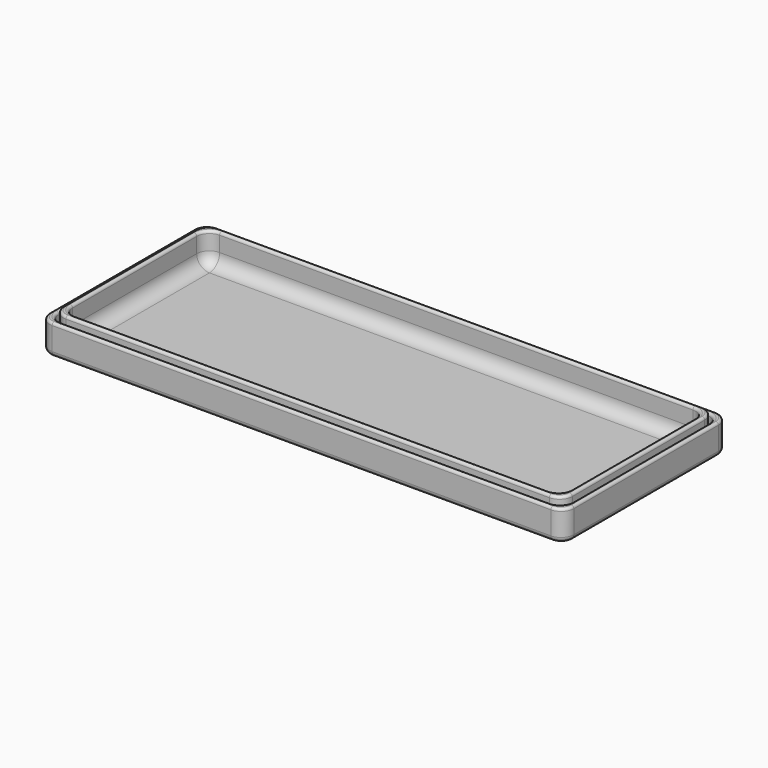
from build123d import *

# Parameters (mm, degrees)
F0_W     = 206
F0_H     = 81
F1_DEPTH = 2
F2_W     = 200
F2_H     = 75
F2_W_2   = 196
F2_H_2   = 71
F3_DEPTH = 12
F2_W_3   = 206
F2_H_3   = 81
F2_W_4   = 202
F2_H_4   = 77
F4_DEPTH = 10
F5_R     = 5
F6_R     = 5
F7_R     = 0.99999
F8_R     = 5
F9_R     = 5
F10_R    = 2
F11_R    = 0.99999
F12_R    = 5


# Not quite as in the source:
# - a fillet or chamfer is up to 0.001 mm smaller than in the source, because OpenCascade refuses the exact size


with BuildPart() as f1:
    # F0 (on Top) → F1 (new body)
    with BuildSketch(Plane.XY):
        Rectangle(F0_W, F0_H)
    extrude(amount=F1_DEPTH)

    # F2 (on face) → F3 (join)
    with BuildSketch(Plane.XY.offset(2)):
        Rectangle(F2_W, F2_H)
        Rectangle(F2_W_2, F2_H_2, mode=Mode.SUBTRACT)
    extrude(amount=F3_DEPTH)

    # F2 (on face) → F4 (join)
    with BuildSketch(Plane.XY.offset(2)):
        Rectangle(F2_W_3, F2_H_3)
        Rectangle(F2_W_4, F2_H_4, mode=Mode.SUBTRACT)
    extrude(amount=F4_DEPTH)

    # F5
    f5_edges = [f1.edges().sort_by_distance(p)[0] for p in [
        (-100, -37.5, 8),
        (-100, 37.5, 8),
        (100, 37.5, 8),
        (100, -37.5, 8),
    ]]
    fillet(f5_edges, radius=F5_R)

    # F6
    f6_edges = [f1.edges().sort_by_distance(p)[0] for p in [
        (-98, -35.5, 8),
        (-98, 35.5, 8),
        (98, 35.5, 8),
        (98, -35.5, 8),
    ]]
    fillet(f6_edges, radius=F6_R)

    # F7 (radius 1 in the source; OpenCascade refuses exactly that, so slightly less here)
    f7_edges = [f1.edges().sort_by_distance(p)[0] for p in [
        (-98, 0, 14),
        (-96.535534, -34.035534, 14),
        (-96.535534, 34.035534, 14),
        (0, -35.5, 14),
        (0, 35.5, 14),
        (96.535534, -34.035534, 14),
        (96.535534, 34.035534, 14),
        (98, 0, 14),
        (0, 37.5, 14),
        (98.535534, 36.035534, 14),
        (-98.535534, 36.035534, 14),
        (100, 0, 14),
        (-100, 0, 14),
        (98.535534, -36.035534, 14),
        (-98.535534, -36.035534, 14),
        (0, -37.5, 14),
    ]]
    fillet(f7_edges, radius=F7_R)

    # F8
    f8_edges = [f1.edges().sort_by_distance(p)[0] for p in [
        (-101, 38.5, 7),
        (-101, -38.5, 7),
        (101, -38.5, 7),
        (101, 38.5, 7),
    ]]
    fillet(f8_edges, radius=F8_R)

    # F9
    f9_edges = [f1.edges().sort_by_distance(p)[0] for p in [
        (-103, -40.5, 6),
        (103, -40.5, 6),
        (103, 40.5, 6),
        (-103, 40.5, 6),
    ]]
    fillet(f9_edges, radius=F9_R)

    # F10
    f10_edges = [f1.edges().sort_by_distance(p)[0] for p in [
        (0, -40.5, 0),
        (-101.535534, -39.035534, 0),
        (101.535534, -39.035534, 0),
        (-103, 0, 0),
        (103, 0, 0),
        (-101.535534, 39.035534, 0),
        (101.535534, 39.035534, 0),
        (0, 40.5, 0),
    ]]
    fillet(f10_edges, radius=F10_R)

    # F11 (radius 1 in the source; OpenCascade refuses exactly that, so slightly less here)
    f11_edges = [f1.edges().sort_by_distance(p)[0] for p in [
        (-103, 0, 12),
        (-101.535534, 39.035534, 12),
        (-101.535534, -39.035534, 12),
        (0, 40.5, 12),
        (0, -40.5, 12),
        (101.535534, 39.035534, 12),
        (101.535534, -39.035534, 12),
        (103, 0, 12),
        (-101, 0, 12),
        (-99.535534, -37.035534, 12),
        (-99.535534, 37.035534, 12),
        (0, -38.5, 12),
        (0, 38.5, 12),
        (99.535534, -37.035534, 12),
        (99.535534, 37.035534, 12),
        (101, 0, 12),
    ]]
    fillet(f11_edges, radius=F11_R)

    # F12
    f12_edges = [f1.edges().sort_by_distance(p)[0] for p in [
        (-98, 0, 2),
        (-96.535534, -34.035534, 2),
        (-96.535534, 34.035534, 2),
        (0, -35.5, 2),
        (0, 35.5, 2),
        (96.535534, -34.035534, 2),
        (96.535534, 34.035534, 2),
        (98, 0, 2),
    ]]
    fillet(f12_edges, radius=F12_R)


solid = f1.part
